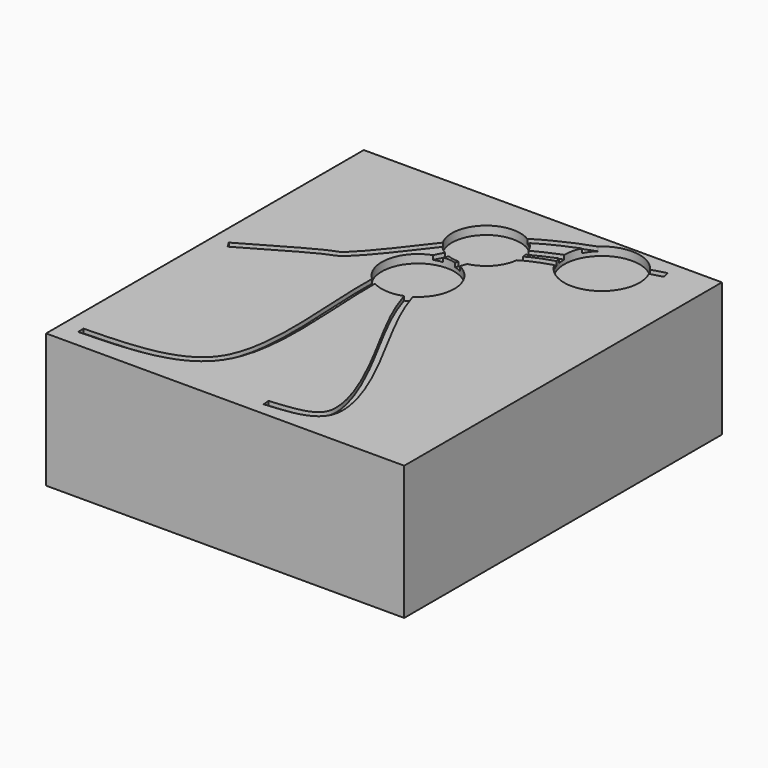
from build123d import *

# Parameters (mm, degrees)
F0_W     = 130.9855282307
F0_H     = 145.2465355396
F1_DEPTH = 49.022
F3_DEPTH = 1.524
F5_R     = 12.5102239431
F5_R_2   = 13.2805824437
F5_R_3   = 13.7943823286
F6_DEPTH = 3.0490001


# Not quite as in the source:
# - the dataset's text gives a spline's control points without its knots; the knots are read off the source's solid


with BuildPart() as f1:
    # F0 (on Top) → F1 (new body)
    with BuildSketch(Plane.XY):
        Rectangle(F0_W, F0_H)
    extrude(amount=F1_DEPTH)

    # F2 (on face) → F3 (cut)
    with BuildSketch(Plane.XY.offset(49.022)):
        with BuildLine():
            add(Edge.make_bspline(
                [(50.4779815674, 64.9829134345), (31.3918715338, 59.5214666512), (-3.487004779, 49.5409558762), (-15.6453692052, 11.9647068929), (-2.1023920017, -64.5705675352), (-41.1428074038, -65.667295936), (-58.9387007058, -66.1672204733)],
                knots=[0, 0, 0, 0, 0.2599325194, 0.4750131995, 0.7606939119, 1, 1, 1, 1], degree=3))
            Line((50.4779815674, 64.9829134345), (49.7792114633, 67.4249042884))
            add(Edge.make_bspline(
                [(49.7792114633, 67.4249042884), (45.1900131596, 66.1117156779), (35.983030947, 63.4773571242), (24.9634393602, 59.8780415923), (16.7675386901, 56.6304273615), (11.0101558036, 53.9599994247), (5.722128972, 50.999624558), (1.775228701, 48.240495565), (-1.0608679889, 45.8212320515), (-3.6598752526, 43.2605938722), (-6.4706701402, 39.7867303312), (-9.1565226266, 35.1677949432), (-11.1885106867, 30.0968099352), (-12.6199051295, 24.5633154421), (-13.5120522291, 18.5393655517), (-13.9286356802, 11.9864732231), (-13.9156859898, 4.8495232235), (-13.6217913492, -2.6996735151), (-13.2125189706, -10.4830511238), (-12.8438573681, -18.3117778755), (-12.6712147373, -25.9899568518), (-12.8461611483, -33.3140199045), (-13.5129916221, -40.0707917022), (-14.799358162, -46.0369508746), (-16.2958904269, -49.7473033512), (-17.5268786948, -51.8505408472), (-18.4109819496, -53.1531931269), (-20.1504783643, -55.2205945797), (-23.1774596577, -57.6419802794), (-27.6790372583, -59.8464863851), (-32.9638612549, -61.424333733), (-38.8903646152, -62.4676454356), (-47.4433084159, -63.3016177177), (-54.3622412157, -63.4976561349), (-59.0100265703, -63.6282223225)],
                knots=[0, 0, 0, 0, 0.0625, 0.125, 0.15625, 0.1875, 0.21875, 0.25, 0.265625, 0.28125, 0.3125, 0.34375, 0.375, 0.40625, 0.4375, 0.46875, 0.5, 0.53125, 0.5625, 0.59375, 0.625, 0.65625, 0.6875, 0.71875, 0.75, 0.7578125, 0.765625, 0.78125, 0.8125, 0.84375, 0.875, 0.90625, 0.9375, 1, 1, 1, 1], degree=3))
            Line((-59.0100265703, -63.6282223225), (-58.9387007058, -66.1672204733))
        make_face()
        with BuildLine():
            add(Edge.make_bspline(
                [(43.3583967388, 55.2403256297), (31.5804766366, 53.5209610847), (10.5799999147, 50.4552691126), (-3.3623011323, 31.2177677669), (3.2116538709, 3.4608221176), (16.455375075, -19.1179344117), (39.2983856182, -65.6550572761), (18.8556702836, -67.3417658966), (10.3835100308, -68.0407956243)],
                knots=[0, 0, 0, 0, 0.1804172127, 0.3216907096, 0.480640078, 0.6548308668, 0.8569501085, 1, 1, 1, 1], degree=3))
            Line((43.3583967388, 55.2403256297), (42.9914913227, 57.7536859799))
            add(Edge.make_bspline(
                [(42.9914913227, 57.7536859799), (38.9113927813, 57.1580649609), (32.7474012883, 56.2593791165), (24.8813840562, 54.6510098535), (19.2617966132, 53.1316846984), (14.8966974415, 51.5064599919), (11.6497438632, 49.9253069569), (8.5854707809, 48.1276237284), (5.1803673082, 45.4849423726), (1.8357329406, 41.7251687151), (-0.6934133152, 37.4314256766), (-2.0693329255, 33.4739130275), (-2.7061314875, 30.1152442293), (-2.9537221071, 27.5393192307), (-2.9979186054, 24.9222932657), (-2.8131896993, 21.3961414394), (-2.1765658932, 16.9520635586), (-1.1208449904, 12.5461908144), (-0.0923178146, 9.0993165954), (0.75504195, 6.5666449222), (1.6610329982, 4.1034092884), (2.9323545553, 0.9168834804), (4.6477739028, -2.9446795524), (6.9173640099, -7.5548556599), (9.4124634081, -12.3238356409), (11.6959879182, -16.5874165957), (13.6564939954, -20.2669439969), (15.1978885073, -23.1868452906), (16.8085852213, -26.2829548632), (18.9920694521, -30.58328251), (21.6917526921, -36.1785867966), (24.5647672607, -42.8932298448), (26.3866599389, -48.18183769), (27.3461511704, -52.0197848006), (27.7830639992, -54.6398848849), (27.8904494301, -56.549229123), (27.8217365879, -57.8728550238), (27.6972357362, -58.7538082068), (27.5056562, -59.5184232545), (27.2599090649, -60.1575444745), (26.9522997672, -60.7195923452), (26.4516381198, -61.401845922), (25.6308984319, -62.1698589289), (24.2656070096, -62.991466468), (22.5246869802, -63.6881816296), (19.770693817, -64.4371129925), (15.6763807594, -65.0550550251), (12.0254347308, -65.3566908769), (10.1746468336, -65.5093975918)],
                knots=[0, 0, 0, 0, 0.0625, 0.09375, 0.125, 0.15625, 0.171875, 0.1875, 0.21875, 0.25, 0.28125, 0.3125, 0.328125, 0.34375, 0.359375, 0.375, 0.40625, 0.4375, 0.453125, 0.46875, 0.484375, 0.5, 0.53125, 0.5625, 0.59375, 0.625, 0.640625, 0.65625, 0.671875, 0.6875, 0.71875, 0.75, 0.78125, 0.796875, 0.8125, 0.828125, 0.8359375, 0.84375, 0.8515625, 0.859375, 0.8671875, 0.875, 0.890625, 0.90625, 0.921875, 0.9375, 0.96875, 1, 1, 1, 1], degree=3))
            Line((10.1746468336, -65.5093975918), (10.3835100308, -68.0407956243))
        make_face()
        with BuildLine():
            add(Edge.make_bspline(
                [(37.1756069362, 67.6059126854), (36.4034325675, 67.8017052724), (33.2831633267, 68.5928809596), (2.4612766181, 58.36687931), (-13.5086405161, 35.3233847923), (-28.9044396572, 16.7967113125), (-33.2948104275, 16.362519406), (-47.885321472, 7.8709997561), (-58.5639849305, 1.6561330995)],
                knots=[0, 0, 0, 0, 0.0717823038, 0.2900641662, 0.5167027384, 0.7025169643, 0.7822748488, 1, 1, 1, 1], degree=3))
            Line((37.1756069362, 67.6059126854), (37.7998936352, 70.0679986868))
            add(Edge.make_bspline(
                [(37.7998936352, 70.0679986868), (37.6318128704, 70.1106172573), (37.2345108972, 70.212494648), (36.4438685228, 70.360258724), (35.4988296217, 70.4347112819), (34.42314464, 70.4057196781), (33.1790788341, 70.2593809818), (31.2948534503, 69.9133655528), (28.4905882211, 69.2178650646), (24.5248049736, 67.9881683237), (20.1390579892, 66.3918573259), (15.5243992251, 64.4571017822), (11.6508060795, 62.5852475766), (8.632261529, 60.9429921553), (6.432476722, 59.6414208028), (4.3208583648, 58.2690787695), (2.3269834306, 56.8407772516), (0.4383733624, 55.3612746485), (-1.9491040976, 53.3270949226), (-4.7106774056, 50.6817158568), (-7.7400856818, 47.3827333849), (-10.560362747, 43.9961644801), (-13.2476486065, 40.555879534), (-15.440300993, 37.6689084256), (-17.2025588007, 35.362758753), (-18.9873344287, 33.0576953937), (-21.2427780654, 30.2071398918), (-23.884452663, 26.9831402297), (-25.9474170316, 24.57998811), (-27.4593981685, 22.9034862391), (-28.5085152317, 21.7894729594), (-29.4547423703, 20.8406635433), (-30.1376876035, 20.2089267758), (-30.6026183532, 19.8139680505), (-30.9991018219, 19.5022796805), (-31.3638637851, 19.261231733), (-31.7184387722, 19.077292264), (-32.1748390659, 18.8901906365), (-32.7439852307, 18.6838436655), (-33.3157355145, 18.4669815143), (-33.8029360056, 18.2716191769), (-34.3397677536, 18.040779885), (-35.0985318858, 17.6964404085), (-36.1438206163, 17.1935083733), (-37.5495282013, 16.480546241), (-39.6167546396, 15.3932046708), (-42.5363841777, 13.7983243881), (-46.4780264607, 11.5791456807), (-52.1739714036, 8.313917437), (-56.7762069958, 5.6354493426), (-59.8416152065, 3.8514149125)],
                knots=[0, 0, 0, 0, 0.015625, 0.03125, 0.046875, 0.0625, 0.078125, 0.09375, 0.125, 0.15625, 0.1875, 0.21875, 0.25, 0.265625, 0.28125, 0.296875, 0.3125, 0.328125, 0.34375, 0.375, 0.40625, 0.4375, 0.46875, 0.5, 0.515625, 0.53125, 0.5625, 0.59375, 0.625, 0.640625, 0.65625, 0.671875, 0.6875, 0.6953125, 0.703125, 0.71875, 0.734375, 0.75, 0.765625, 0.7734375, 0.78125, 0.7890625, 0.796875, 0.8125, 0.828125, 0.84375, 0.875, 0.90625, 0.9375, 1, 1, 1, 1], degree=3))
            Line((-59.8416152065, 3.8514149125), (-58.5639849305, 1.6561330995))
        make_face()
    extrude(amount=-F3_DEPTH, mode=Mode.SUBTRACT)

    # F5 (on face) → F6 (cut, through all)
    with BuildSketch(Plane.XY.offset(45.974)):
        with Locations((-1.2250904692, 48.2072196901)):
            Circle(F5_R)
        with Locations((-4.93457634, 21.7108931392)):
            Circle(F5_R_2)
        with Locations((33.4850996733, 57.7536859799)):
            Circle(F5_R_3)
    extrude(amount=F6_DEPTH, mode=Mode.SUBTRACT)


solid = f1.part
